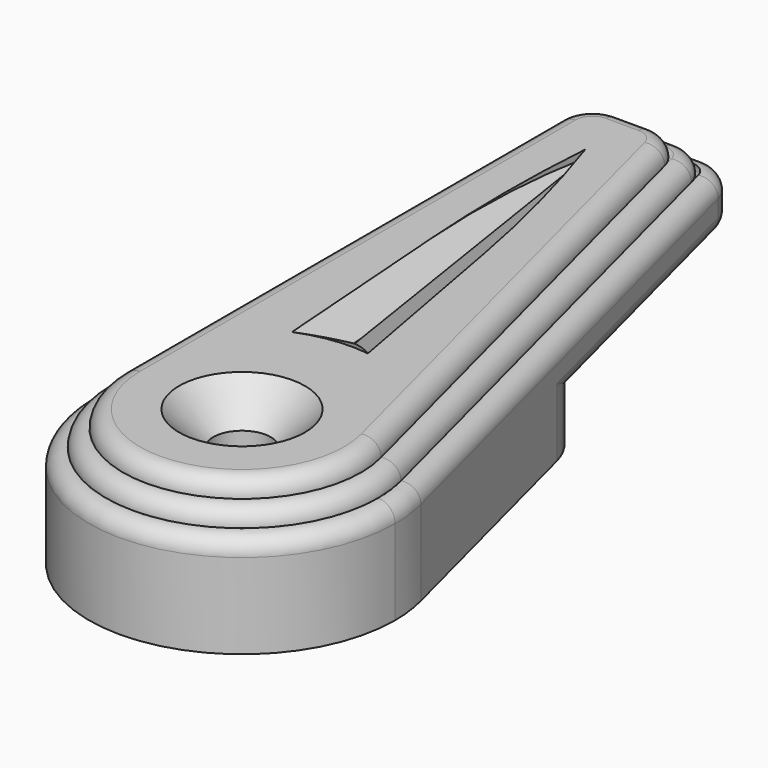
from build123d import *

# Parameters (mm, degrees)
F0_W          = 2.5
F0_H          = 2.5
F1_DEPTH      = 3
F2_R          = 0.85
F3_DEPTH      = 1
F2_W          = 2.5
F2_H          = 2.5
F4_DEPTH      = 1
F5_R          = 1
F6_DEPTH      = 0.5
F7_R          = 1
F8_W          = 8
F8_H          = 1.5
F9_DEPTH      = 25
F10_R         = 2
F11_R         = 0.49999
F12_SIZE      = 0.99999
F14_DEPTH     = 0.5
F15_T4_DEPTH  = 20.2776635659
F15_S5_R      = 4
F15_T6_DEPTH  = 12
F15_S7_R      = 38.7980814883
F15_T8_DEPTH  = 12
F15_T12_DEPTH = 20.3291293813
F15_S13_R     = 4
F15_T14_DEPTH = 12
F15_S15_R     = 40.0741234766
F15_T16_DEPTH = 12
F15_T20_ANGLE = 99.6095230311


# Not quite as in the source:
# - a fillet or chamfer that OpenCascade refuses, or shapes differently, is made with other operations: its cross-section is extruded or revolved along the edge and cut away or added
# - a fillet or chamfer is up to 0.001 mm smaller than in the source, because OpenCascade refuses the exact size


with BuildPart() as f1:
    # F0 (on Top) → F1 (new body)
    with BuildSketch(Plane.XY):
        with BuildLine():
            ThreePointArc((-4.5, 0), (0, -4.5), (4.5, 0))
            ThreePointArc((4.5, 0), (4.4641336332, 0.5670193162), (4.3571062645, 1.125))
            ThreePointArc((4.3571062645, 1.125), (-0.5670193162, 4.4641336332), (-4.5, 0))
        make_face()
        Rectangle(F0_W, F0_H, mode=Mode.SUBTRACT)
        with BuildLine():
            ThreePointArc((-4.5, 0), (-0.5670193162, 4.4641336332), (4.3571062645, 1.125))
            Line((4.3571062645, 1.125), (0, 18))
            Line((0, 18), (-4.5, 18))
            Line((-4.5, 18), (-4.5, 0))
        make_face()
    extrude(amount=F1_DEPTH)

    # F2 (on face) → F3 (join)
    with BuildSketch(Plane.XY.offset(3)):
        with BuildLine():
            Line((-3.5, 17), (-3.5, 0))
            ThreePointArc((-3.5, 0), (0.4410150237, -3.4721039369), (3.3888604279, 0.875))
            Line((3.3888604279, 0.875), (-0.7745966692, 17))
            Line((-0.7745966692, 17), (-3.5, 17))
        make_face()
        Circle(F2_R, mode=Mode.SUBTRACT)
    extrude(amount=-F3_DEPTH)

    # F2 (on face) → F4 (join)
    with BuildSketch(Plane.XY.offset(3)):
        with BuildLine():
            Line((-3.5, 17), (-3.5, 0))
            ThreePointArc((-3.5, 0), (0.4410150237, -3.4721039369), (3.3888604279, 0.875))
            Line((3.3888604279, 0.875), (-0.7745966692, 17))
            Line((-0.7745966692, 17), (-3.5, 17))
        make_face()
        Rectangle(F2_W, F2_H, mode=Mode.SUBTRACT)
        Rectangle(F2_W, F2_H)
        Circle(F2_R, mode=Mode.SUBTRACT)
    extrude(amount=F4_DEPTH)

    # F5 (on face) → F6 (join)
    with BuildSketch(Plane.XY.offset(3)):
        with BuildLine():
            Line((3.8729833462, 1), (-0.3872983346, 17.5))
            Line((-0.3872983346, 17.5), (-4, 17.5))
            Line((-4, 17.5), (-4, 0))
            ThreePointArc((-4, 0), (0.5040171699, -3.9681187851), (3.8729833462, 1))
        make_face()
        Circle(F5_R, mode=Mode.SUBTRACT)
    extrude(amount=F6_DEPTH)

    # F7
    f7_edges = [f1.edges().sort_by_distance(p)[0] for p in [
        (-4.5, 18, 1.5),
        (0, 18, 1.5),
        (-4, 17.5, 3.25),
        (-3.5, 17, 3.75),
        (-0.387298, 17.5, 3.25),
        (-0.774597, 17, 3.75),
    ]]
    fillet(f7_edges, radius=F7_R)

    # F8 (on face) → F9 (cut)
    with BuildSketch(Plane(origin=(-4.5, 0, 0), x_dir=(0, -1, 0), z_dir=(-1, 0, 0))):
        with Locations((-14, 0.75)):
            Rectangle(F8_W, F8_H)
    extrude(amount=-F9_DEPTH, mode=Mode.SUBTRACT)

    # F10
    f10_edges = [f1.edges().sort_by_distance(p)[0] for p in [
        (2.065591, 10, 0.75),
        (-4.5, 10, 0.75),
    ]]
    fillet(f10_edges, radius=F10_R)

    # F11 (radius 0.5 in the source; OpenCascade refuses exactly that, so slightly less here)
    f11_edges = [f1.edges().sort_by_distance(p)[0] for p in [
        (1.12962, 13.625, 1.5),
        (2.275378, 9.1875, 3),
        (1.839667, 8.875, 3.5),
        (1.403956, 8.5625, 4),
        (-4.5, 8.5, 3),
        (-4.5, 13.5, 1.5),
        (0.567019, -4.464134, 3),
        (-4.207107, 17.707107, 1.5),
        (-0.162224, 17.790569, 1.5),
        (-2.137298, 18, 1.5),
        (-4.207107, 17.707107, 3),
        (-2.137298, 18, 3),
        (-0.162224, 17.790569, 3),
        (-0.549523, 17.290569, 3.5),
        (0.504017, -3.968119, 3.5),
        (-2.080948, 17.5, 3.5),
        (-4, 8.25, 3.5),
        (-3.707107, 17.207107, 3.5),
        (-0.936821, 16.790569, 4),
        (0.441015, -3.472104, 4),
        (-2.024597, 17, 4),
        (-3.5, 8, 4),
        (-3.207107, 16.707107, 4),
    ]]
    fillet(f11_edges, radius=F11_R)

    # F12 (size 1 in the source; OpenCascade refuses exactly that, so slightly less here)
    f12_edges = [f1.edges().sort_by_distance(p)[0] for p in [
        (-0.85, 0, 4),
    ]]
    chamfer(f12_edges, length=F12_SIZE)

    # F13 (on face) → F14 (cut)
    with BuildSketch(Plane.XY.offset(4)):
        with BuildLine():
            Line((-1.9118950039, 9.3540496218), (-1.5, 3.7080992435))
            ThreePointArc((-1.5, 3.7080992435), (-0.5040171699, 3.9681187851), (0.5253439439, 3.9653516541))
            Line((0.5253439439, 3.9653516541), (-0.487328028, 9.482675827))
            ThreePointArc((-0.487328028, 9.482675827), (-1.1014215296, 12.266690459), (-1.9118950039, 15))
            ThreePointArc((-1.9118950039, 15), (-2.0147321041, 12.1770248109), (-1.9118950039, 9.3540496218))
        make_face()
    extrude(amount=-F14_DEPTH, mode=Mode.SUBTRACT)

    # F15: chamfer of 0.5 x 0.9443356708 on 5 edges, made by hand


with BuildPart() as f15_tool2:
    # F15_s3 → F15_t4 (new body)
    with BuildSketch(Plane(origin=(-0.2456386094, 1.3383088255, 0), x_dir=(0, 0, 1), z_dir=(-0.1805283712, 0.9835697775, 0))):
        Polygon((4, 1.2325709013), (3.5, 0.2882352305), (3.5, 1.2325709013), align=None)
    extrude(amount=F15_T4_DEPTH)

    # F15_s5 → F15_t6 (cut, symmetric)
    with BuildSketch(Plane.XY.offset(3.8)):
        Circle(F15_S5_R)
    extrude(amount=F15_T6_DEPTH, both=True, mode=Mode.SUBTRACT)

    # F15_s7 → F15_t8 (intersect, symmetric)
    with BuildSketch(Plane.XY.offset(3.8)):
        with Locations((36.7833493842, 12.1770248109)):
            Circle(F15_S7_R)
    extrude(amount=F15_T8_DEPTH, both=True, mode=Mode.INTERSECT)


with BuildPart() as f1_1:
    add(f1.part)

    # F15_t1: union F15_tool2
    add(f15_tool2.part)


with BuildPart() as f15_tool10:
    # F15_s11 → F15_t12 (new body)
    with BuildSketch(Plane(origin=(-1.5783136418, 21.6343495778, 0), x_dir=(0, 0, 1), z_dir=(0.0727606902, -0.9973494282, 0))):
        Polygon((3.5, 0.2818846111), (4, 1.2262202819), (3.5, 1.2262202819), align=None)
    extrude(amount=F15_T12_DEPTH)

    # F15_s13 → F15_t14 (cut, symmetric)
    with BuildSketch(Plane.XY.offset(3.8)):
        Circle(F15_S13_R)
    extrude(amount=F15_T14_DEPTH, both=True, mode=Mode.SUBTRACT)

    # F15_s15 → F15_t16 (intersect, symmetric)
    with BuildSketch(Plane.XY.offset(3.8)):
        with Locations((-39.9030247393, 2.2481595898)):
            Circle(F15_S15_R)
    extrude(amount=F15_T16_DEPTH, both=True, mode=Mode.INTERSECT)


with BuildPart() as f1_2:
    add(f1_1.part)

    # F15_t9: union F15_tool10
    add(f15_tool10.part)


with BuildPart() as f15_tool18:
    # F15_s19 → F15_t20 (revolve)
    with BuildSketch(Plane(origin=(0, 0, 0), x_dir=(0, 0, 1), z_dir=(-0.5440018863, -0.8390839933, 0))):
        Polygon((3.5, 4.9443356708), (4, 4), (3.5, 4), align=None)
    revolve(axis=Axis((0, 0, 3.5), (0, 0, -1)), revolution_arc=F15_T20_ANGLE)

    split(bisect_by=Plane(origin=(1.2123194871, 0.2225140172, 0), x_dir=(0, 0, 1), z_dir=(-0.9835697775, -0.1805283712, 0)), keep=Keep.TOP)

    split(bisect_by=Plane(origin=(-1.222970097, -0.0892206341, 0), x_dir=(0, 0, 1), z_dir=(0.9973494282, 0.0727606902, 0)), keep=Keep.TOP)


with BuildPart() as f1_3:
    add(f1_2.part)

    # F15_t17: union F15_tool18
    add(f15_tool18.part)


solid = f1_3.part
